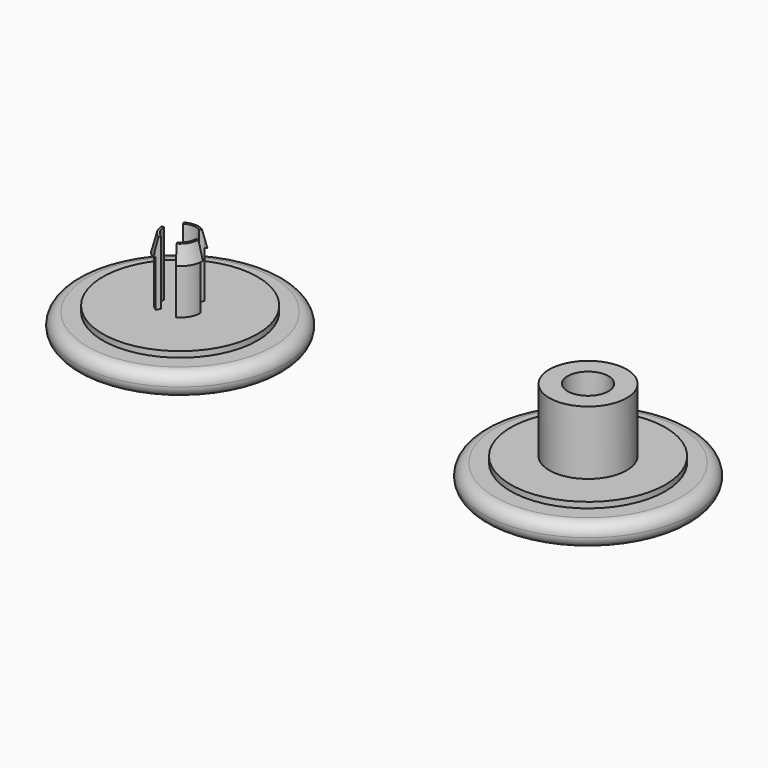
from build123d import *

# Parameters (mm, degrees)
F0_R      = 11.5
F0_R_2    = 8.5
F1_DEPTH  = 2.54
F0_R_3    = 4.25
F2_DEPTH  = 3.175
F3_DEPTH  = 10.175
F4_R      = 1.26999
F5_R      = 11.5
F5_R_2    = 8.5
F6_DEPTH  = 2.54
F5_R_3    = 2.5
F7_DEPTH  = 3.175
F8_DEPTH  = 10.175
F9_R      = 2.25
F10_DEPTH = 7
F11_R     = 1.26999
F12_R     = 2.55
F13_DEPTH = 2
F16_R     = 1.75
F17_DEPTH = 7
F19_DEPTH = 25.4


# Not quite as in the source:
# - a fillet or chamfer is up to 0.001 mm smaller than in the source, because OpenCascade refuses the exact size


with BuildPart() as f1:
    # F0 (on Top) → F1 (new body)
    with BuildSketch(Plane.XY):
        Circle(F0_R)
        Circle(F0_R_2, mode=Mode.SUBTRACT)
    extrude(amount=F1_DEPTH)

    # F0 (on Top) → F2 (join)
    with BuildSketch(Plane.XY):
        Circle(F0_R_2)
        Circle(F0_R_3, mode=Mode.SUBTRACT)
    extrude(amount=F2_DEPTH)

    # F0 (on Top) → F3 (join)
    with BuildSketch(Plane.XY):
        Circle(F0_R_3)
    extrude(amount=F3_DEPTH)

    # F4 (radius 1.27 in the source; OpenCascade refuses exactly that, so slightly less here)
    f4_edges = [f1.edges().sort_by_distance(p)[0] for p in [
        (-11.5, 0, 2.54),
        (-11.5, 0, 0),
    ]]
    fillet(f4_edges, radius=F4_R)

    # F9 (on face) → F10 (cut)
    with BuildSketch(Plane.XY.offset(10.175)):
        Circle(F9_R)
    extrude(amount=-F10_DEPTH, mode=Mode.SUBTRACT)

    # F12 (on face) → F13 (cut)
    with BuildSketch(Plane.XY.offset(3.175)):
        Circle(F12_R)
    extrude(amount=F13_DEPTH, mode=Mode.SUBTRACT)


with BuildPart() as f6:
    # F5 (on Top) → F6 (new body)
    with BuildSketch(Plane.XY):
        with Locations((-44.7985892718, 0)):
            Circle(F5_R)
        with Locations((-44.7985892718, 0)):
            Circle(F5_R_2, mode=Mode.SUBTRACT)
    extrude(amount=F6_DEPTH)

    # F5 (on Top) → F7 (join)
    with BuildSketch(Plane.XY):
        with Locations((-44.7985892718, 0)):
            Circle(F5_R_2)
        with Locations((-44.7985892718, 0)):
            Circle(F5_R_3, mode=Mode.SUBTRACT)
    extrude(amount=F7_DEPTH)

    # F5 (on Top) → F8 (join)
    with BuildSketch(Plane.XY):
        with Locations((-44.7985892718, 0)):
            Circle(F5_R_3)
    extrude(amount=F8_DEPTH)

    # F11 (radius 1.27 in the source; OpenCascade refuses exactly that, so slightly less here)
    f11_edges = [f6.edges().sort_by_distance(p)[0] for p in [
        (-56.298589, 0, 2.54),
        (-56.298589, 0, 0),
    ]]
    fillet(f11_edges, radius=F11_R)

    # F14 (on Front) → F15 (revolve, cut)
    with BuildSketch(Plane.XZ):
        Polygon((-42.5485892718, 8.275), (-42.5485892718, 3.175), (-41.8997183442, 3.175), (-41.6368916631, 8.275), (-42.2985892718, 8.275), align=None)
        Polygon((-42.5485892718, 10.175), (-42.7985892718, 10.175), (-42.2985892718, 8.275), (-41.6368916631, 8.275), (-41.8774240868, 10.2633112086), align=None)
    revolve(axis=Axis((-44.7985892718, 0, 5.0875), (0, 0, 1)), mode=Mode.SUBTRACT)

    # F16 (on face) → F17 (cut)
    with BuildSketch(Plane.XY.offset(10.175)):
        with Locations((-44.7985892718, 0)):
            Circle(F16_R)
    extrude(amount=-F17_DEPTH, mode=Mode.SUBTRACT)

    # F18 (on face) → F19 (cut)
    with BuildSketch(Plane.XY.offset(3.175)):
        with BuildLine():
            Line((-45.9235892718, 1.9485571585), (-47.2724906726, 4.2849229191))
            ThreePointArc((-47.2724906726, 4.2849229191), (-49.0835121909, 2.4739014008), (-49.7463920734, 0))
            Line((-49.7463920734, 0), (-47.0485892718, 0))
            ThreePointArc((-47.0485892718, 0), (-46.7471464303, 1.125), (-45.9235892718, 1.9485571585))
        make_face()
        with BuildLine():
            Line((-47.0485892718, 0), (-44.7985892718, 0))
            Line((-44.7985892718, 0), (-45.9235892718, 1.9485571585))
            ThreePointArc((-45.9235892718, 1.9485571585), (-46.7471464303, 1.125), (-47.0485892718, 0))
        make_face()
        with BuildLine():
            Line((-42.5485892718, 0), (-39.8507864702, 0))
            ThreePointArc((-39.8507864702, 0), (-40.5136663527, 2.4739014008), (-42.324687871, 4.2849229191))
            Line((-42.324687871, 4.2849229191), (-43.6735892718, 1.9485571585))
            ThreePointArc((-43.6735892718, 1.9485571585), (-42.8500321132, 1.125), (-42.5485892718, 0))
        make_face()
        with BuildLine():
            Line((-44.7985892718, 0), (-42.5485892718, 0))
            ThreePointArc((-42.5485892718, 0), (-42.8500321132, 1.125), (-43.6735892718, 1.9485571585))
            Line((-43.6735892718, 1.9485571585), (-44.7985892718, 0))
        make_face()
        with BuildLine():
            ThreePointArc((-47.2724906726, -4.2849229191), (-44.7985892718, -4.9478028016), (-42.324687871, -4.2849229191))
            Line((-42.324687871, -4.2849229191), (-43.6735892718, -1.9485571585))
            ThreePointArc((-43.6735892718, -1.9485571585), (-44.7985892718, -2.25), (-45.9235892718, -1.9485571585))
            Line((-45.9235892718, -1.9485571585), (-47.2724906726, -4.2849229191))
        make_face()
        with BuildLine():
            Line((-43.6735892718, -1.9485571585), (-44.7985892718, 0))
            Line((-44.7985892718, 0), (-45.9235892718, -1.9485571585))
            ThreePointArc((-45.9235892718, -1.9485571585), (-44.7985892718, -2.25), (-43.6735892718, -1.9485571585))
        make_face()
    extrude(amount=F19_DEPTH, mode=Mode.SUBTRACT)


solid = Compound([f1.part, f6.part])
